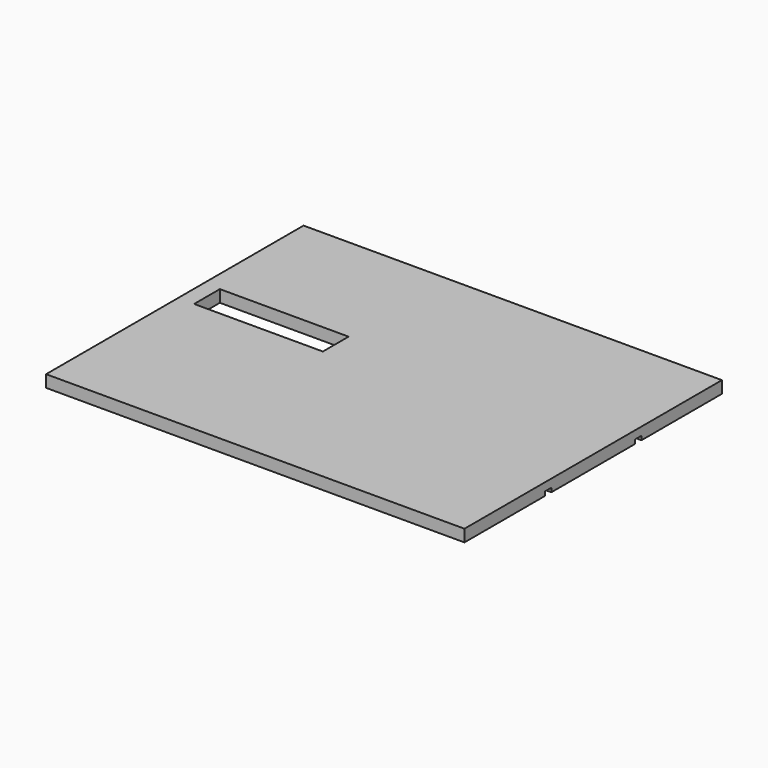
from build123d import *

# Parameters (mm, degrees)
F0_W     = 203.2
F0_H     = 50.8
F1_DEPTH = 19.05
F2_W     = 660.4
F2_H     = 12.699998945
F2_H_2   = 12.6999986589
F3_DEPTH = 6.35


# Not quite as in the source:
# - a feature names something its author has since deleted; it is built from what else it names


with BuildPart() as f1:
    # F0 (on Top) → F1 (new body)
    with BuildSketch(Plane.XY):
        Polygon((614.0642432213, 447.3863640726), (-46.3357567787, 447.3863640726), (-46.3357567787, -60.6136359274), (614.0642432213, -60.6136359274), (614.0642432213, -28.8636359274), (614.0642432213, -9.8136359274), (614.0642432213, 396.5863640726), (614.0642432213, 415.6363640726), align=None)
        with Locations((80.6642432213, 225.1363640726)):
            Rectangle(F0_W, F0_H, mode=Mode.SUBTRACT)
    extrude(amount=F1_DEPTH)

    # F2 (on face) → F3 (cut)
    with BuildSketch(Plane(origin=(0, 0, 0), x_dir=(1, 0, 0), z_dir=(0, 0, -1))):
        with Locations((283.8642432213, -282.2863646001)):
            Rectangle(F2_W, F2_H)
        with Locations((283.8642432213, -104.4863647431)):
            Rectangle(F2_W, F2_H_2)
    extrude(amount=-F3_DEPTH, mode=Mode.SUBTRACT)


solid = f1.part
